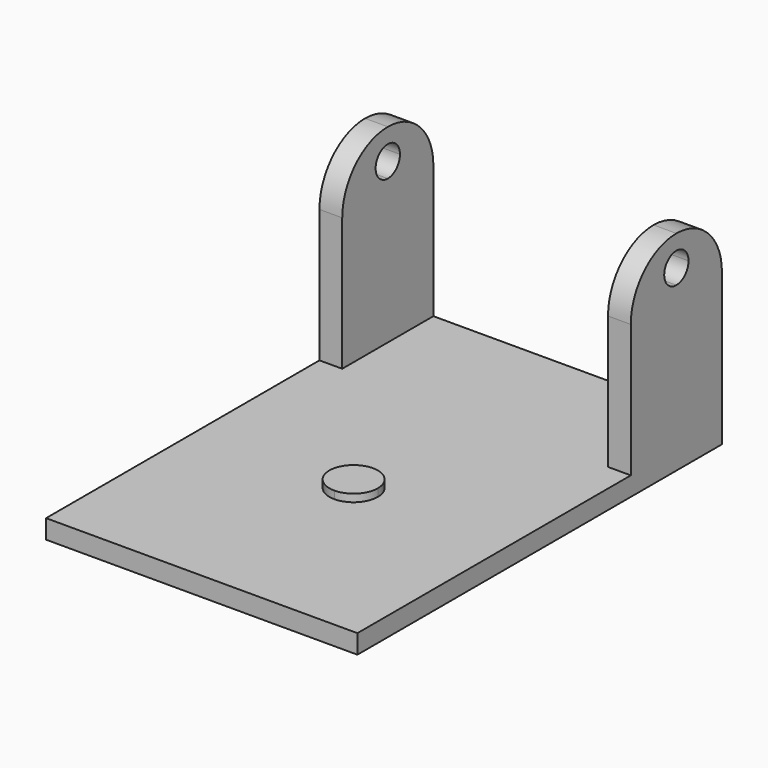
from build123d import *

# Parameters (mm, degrees)
F0_W     = 82
F0_H     = 120
F1_DEPTH = 5
F3_DEPTH = 2
F4_W     = 6
F4_H     = 30
F5_DEPTH = 50
F7_DEPTH = 82.001
F8_R     = 14.99999


# Not quite as in the source:
# - a fillet or chamfer is up to 0.001 mm smaller than in the source, because OpenCascade refuses the exact size


with BuildPart() as f1:
    # F0 (on Top) → F1 (new body)
    with BuildSketch(Plane.XY):
        with Locations((-1.9225833714, 0.167620076)):
            Rectangle(F0_W, F0_H)
    extrude(amount=F1_DEPTH)

    # F2 (on face) → F3 (join)
    with BuildSketch(Plane.XY.offset(5)):
        with BuildLine():
            ThreePointArc((-1.9225833714, -16.2103295776), (2.5873080787, -14.3422713741), (4.4553662822, -9.832379924))
            ThreePointArc((4.4553662822, -9.832379924), (-6.4324748215, -5.3224884739), (-1.9225833714, -16.2103295776))
        make_face()
    extrude(amount=F3_DEPTH)

    # F4 (on face) → F5 (join)
    with BuildSketch(Plane.XY.offset(5)):
        with Locations((-39.9225833714, 45.167620076)):
            Rectangle(F4_W, F4_H)
        with Locations((36.0774166286, 45.167620076)):
            Rectangle(F4_W, F4_H)
    extrude(amount=F5_DEPTH)

    # F6 (on face) → F7 (cut, through all)
    with BuildSketch(Plane.YZ.offset(39.0774166286)):
        with BuildLine():
            Line((45.167620076, 43), (45.167620076, 51))
            ThreePointArc((45.167620076, 51), (41.167620076, 47), (45.167620076, 43))
        make_face()
        with BuildLine():
            ThreePointArc((45.167620076, 43), (47.9960472007, 44.1715728753), (49.167620076, 47))
            ThreePointArc((49.167620076, 47), (47.9960472007, 49.8284271247), (45.167620076, 51))
            Line((45.167620076, 51), (45.167620076, 43))
        make_face()
    extrude(amount=-F7_DEPTH, mode=Mode.SUBTRACT)

    # F8 (radius 15 in the source; OpenCascade refuses exactly that, so slightly less here)
    f8_edges = [f1.edges().sort_by_distance(p)[0] for p in [
        (36.077417, 30.16762, 55),
        (-39.922583, 30.16762, 55),
        (-39.922583, 60.16762, 55),
        (36.077417, 60.16762, 55),
    ]]
    fillet(f8_edges, radius=F8_R)


solid = f1.part
